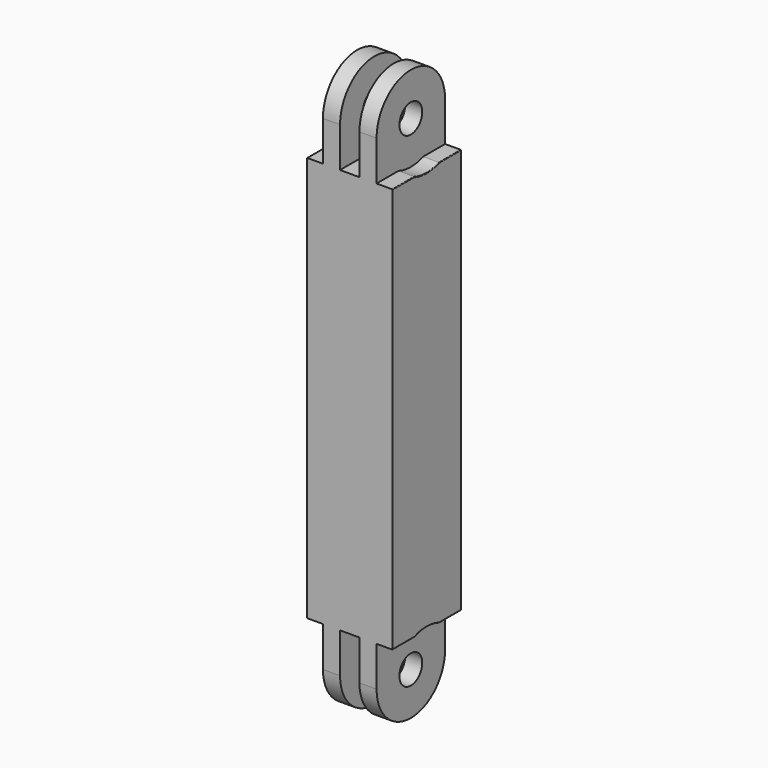
from build123d import *

# Parameters (mm, degrees)
F1_R         = 2.5
F2_DEPTH     = 7.5
F3_W         = 3.4
F3_H         = 15.4505071864
F3_W_2       = 3.8797123611
F3_W_3       = 3.8316924378
F4_DEPTH     = 16.41578
F6_DEPTH     = 2.8
F8_DEPTH     = 2.8
F9_R         = 0.1
F10_R        = 2.5
F11_DEPTH    = 7.5
F12_W        = 3
F12_H        = 7.5577301905
F13_DEPTH    = 15.0010001
F14_T1_DEPTH = 16.5892781094
F16_W        = 15
F16_H        = 15
F17_DEPTH    = 30


# Not quite as in the source:
# - a fillet or chamfer that OpenCascade refuses, or shapes differently, is made with other operations: its cross-section is extruded or revolved along the edge and cut away or added


with BuildPart() as f2:
    # F1 (on Right) → F2 (new body, symmetric)
    with BuildSketch(Plane.YZ):
        with BuildLine():
            Line((7.5, -12.5), (7.5, 0))
            ThreePointArc((7.5, 0), (0, 7.5), (-7.5, 0))
            Line((-7.5, 0), (-7.5, -12.5))
            Line((-7.5, -12.5), (7.5, -12.5))
        make_face()
        Circle(F1_R, mode=Mode.SUBTRACT)
    extrude(amount=F2_DEPTH, both=True)

    # F3 (on Front) → F4 (cut, symmetric)
    with BuildSketch(Plane.XZ):
        with Locations((0, 0.7252535932)):
            Rectangle(F3_W, F3_H)
        with Locations((-6.6398561805, 0.7252535932)):
            Rectangle(F3_W_2, F3_H)
        with Locations((6.6158462189, 0.7252535932)):
            Rectangle(F3_W_3, F3_H)
    extrude(amount=F4_DEPTH, both=True, mode=Mode.SUBTRACT)

    # F5 (on face) → F6 (cut, through all)
    with BuildSketch(Plane(origin=(-7.5, 0, 0), x_dir=(0, -1, 0), z_dir=(-1, 0, 0))):
        with BuildLine():
            ThreePointArc((2.6925824036, -7), (6.1824092402, -4.2459175671), (7.5, 0))
            ThreePointArc((7.5, 0), (-4.2459175671, 6.1824092402), (-2.6925824036, -7))
            Line((-2.6925824036, -7), (2.6925824036, -7))
        make_face()
        with BuildLine():
            Line((2.6925824036, -7), (-2.6925824036, -7))
            ThreePointArc((-2.6925824036, -7), (0, -7.5), (2.6925824036, -7))
        make_face()
    extrude(amount=-F6_DEPTH, mode=Mode.SUBTRACT)

    # F7 (on face) → F8 (cut, through all)
    with BuildSketch(Plane.YZ.offset(7.5)):
        with BuildLine():
            Line((2.6925824036, -7), (-2.6925824036, -7))
            ThreePointArc((-2.6925824036, -7), (0, -7.5), (2.6925824036, -7))
        make_face()
        with BuildLine():
            ThreePointArc((2.6925824036, -7), (6.1824092402, -4.2459175671), (7.5, 0))
            ThreePointArc((7.5, 0), (-4.2459175671, 6.1824092402), (-2.6925824036, -7))
            Line((-2.6925824036, -7), (2.6925824036, -7))
        make_face()
    extrude(amount=-F8_DEPTH, mode=Mode.SUBTRACT)

    # F9
    f9_edges = [f2.edges().sort_by_distance(p)[0] for p in [
        (7.5, -5.096291, -7),
        (7.5, 0, -7.5),
        (7.5, 5.096291, -7),
        (-7.5, 5.096291, -7),
        (-7.5, 0, -7.5),
        (-7.5, -5.096291, -7),
    ]]
    fillet(f9_edges, radius=F9_R)

    # F16 (on face) → F17 (join)
    with BuildSketch(Plane(origin=(0, 0, -12.5), x_dir=(1, 0, 0), z_dir=(0, 0, -1))):
        Rectangle(F16_W, F16_H)
    extrude(amount=F17_DEPTH)

    # F18: F2 across face


with BuildPart() as f11:
    # F10 (on Right) → F11 (new body, symmetric)
    with BuildSketch(Plane.YZ):
        with BuildLine():
            Line((-7.5, 15.0892781094), (-7.5, 0))
            ThreePointArc((-7.5, 0), (0, -7.5), (7.5, 0))
            Line((7.5, 0), (7.5, 15.0892781094))
            Line((7.5, 15.0892781094), (-7.5, 15.0892781094))
        make_face()
        Circle(F10_R, mode=Mode.SUBTRACT)
    extrude(amount=F11_DEPTH, both=True)

    # F12 (on face) → F13 (cut, through all)
    with BuildSketch(Plane.XZ.offset(7.5)):
        with Locations((-3.2, 3.7788650952)):
            Rectangle(F12_W, F12_H)
        with Locations((3.2, 3.7788650952)):
            Rectangle(F12_W, F12_H)
    extrude(amount=-F13_DEPTH, mode=Mode.SUBTRACT)

    # F14: fillet of radius 0.1 on 4 edges, made by hand

    # F14_s2 → F14_t1 (cut)
    with BuildSketch(Plane.XY.offset(-1.25)):
        with BuildLine():
            ThreePointArc((-7.4, 7.5), (-7.4707106781, 7.4707106781), (-7.5, 7.4))
            Line((-7.5, 7.4), (-7.5, 7.5))
            Line((-7.5, 7.5), (-7.4, 7.5))
        make_face()
        with BuildLine():
            ThreePointArc((-7.5, -7.4), (-7.4707106781, -7.4707106781), (-7.4, -7.5))
            Line((-7.4, -7.5), (-7.5, -7.5))
            Line((-7.5, -7.5), (-7.5, -7.4))
        make_face()
        with BuildLine():
            ThreePointArc((7.4, 7.5), (7.4707106781, 7.4707106781), (7.5, 7.4))
            Line((7.5, 7.4), (7.5, 7.5))
            Line((7.5, 7.5), (7.4, 7.5))
        make_face()
        with BuildLine():
            ThreePointArc((7.5, -7.4), (7.4707106781, -7.4707106781), (7.4, -7.5))
            Line((7.4, -7.5), (7.5, -7.5))
            Line((7.5, -7.5), (7.5, -7.4))
        make_face()
    extrude(amount=F14_T1_DEPTH, mode=Mode.SUBTRACT)


with BuildPart() as f2_1:
    add(f2.part)
    add(f2.part.mirror(Plane(origin=(0, 0, -42.5), x_dir=(1, 0, 0), z_dir=(0, 0, -1))))


solid = f2_1.part
